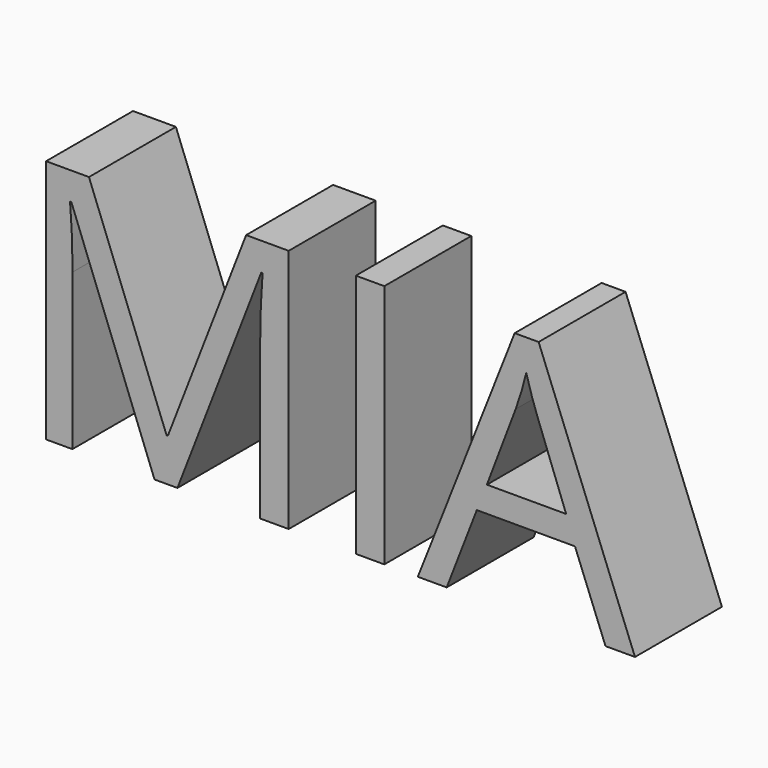
from build123d import *

# Parameters (mm, degrees)
F0_TEXT_SIZE = 80.1912250204
F1_DEPTH     = 12.7


# Not quite as in the source:
# - Text() gives the source's letters only with a copy of the font that has no kerning and outlines rounded to 1/6400 em; it was checked with that copy


with BuildPart() as f1:
    # F0 (on Front) → F1 (new body, symmetric)
    with BuildSketch(Plane.XZ):
        with Locations((-27.834450826, 0)):
            Text('MIA', F0_TEXT_SIZE, font='Open Sans', text_align=(TextAlign.LEFT, TextAlign.BOTTOM))
    extrude(amount=F1_DEPTH, both=True)


solid = f1.part
